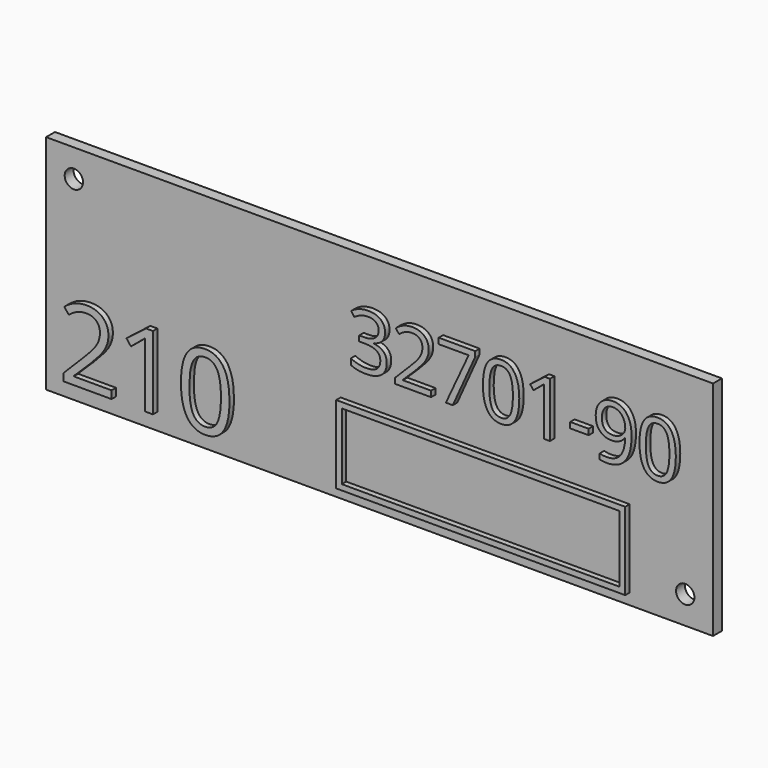
from build123d import *

# Parameters (mm, degrees)
F0_W         = 120
F0_H         = 40
F1_DEPTH     = 2
F3_D         = 3.3
F4_TEXT_SIZE = 13.8283697648
F5_DEPTH     = 1
F6_TEXT_SIZE = 18.4937691891
F7_DEPTH     = 1
F8_W         = 52
F8_H         = 14
F8_W_2       = 49.99999962
F8_H_2       = 11.99999962
F9_DEPTH     = 1


# Not quite as in the source:
# - Text() gives the source's letters only with a copy of the font that has no kerning and outlines rounded to 1/6400 em; it was checked with that copy


with BuildPart() as f1:
    # F0 (on Front) → F1 (new body)
    with BuildSketch(Plane.XZ):
        Rectangle(F0_W, F0_H)
    extrude(amount=F1_DEPTH)

    # F3 (through all)
    with Locations(Plane.XZ.offset(2)):
        with Locations((-55, 15), (55, -15)):
            Hole(F3_D / 2)

    # F4 (on face) → F5 (join)
    with BuildSketch(Plane.XZ.offset(2)):
        with Locations((-5, 2)):
            Text('32701-90', F4_TEXT_SIZE, font='Open Sans', text_align=(TextAlign.LEFT, TextAlign.BOTTOM))
    extrude(amount=F5_DEPTH)

    # F6 (on face) → F7 (join)
    with BuildSketch(Plane.XZ.offset(2)):
        with Locations((-57, -17)):
            Text('210', F6_TEXT_SIZE, font='Open Sans', text_align=(TextAlign.LEFT, TextAlign.BOTTOM))
    extrude(amount=F7_DEPTH)

    # F8 (on face) → F9 (join)
    with BuildSketch(Plane.XZ.offset(2)):
        with Locations((19, -11)):
            Rectangle(F8_W, F8_H)
        with Locations((19, -11)):
            Rectangle(F8_W_2, F8_H_2, mode=Mode.SUBTRACT)
    extrude(amount=F9_DEPTH)


solid = f1.part
